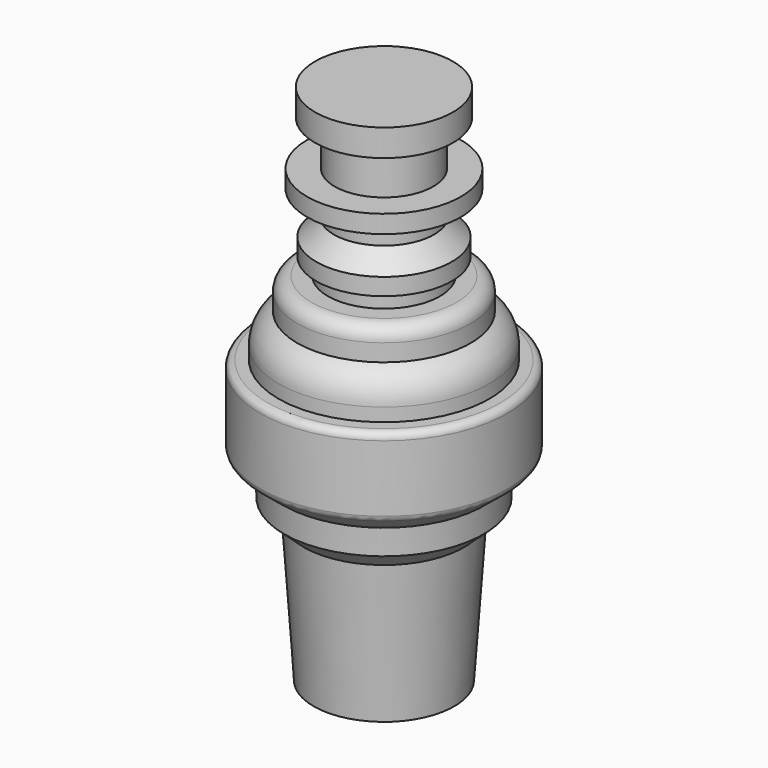
from build123d import *

# Parameters (mm, degrees)
F2_R = 12.7
F4_R = 6.35


# Not quite as in the source:
# - a fillet or chamfer that OpenCascade refuses, or shapes differently, is made with other operations: its cross-section is extruded or revolved along the edge and cut away or added


with BuildPart() as f1:
    # F0 (on Front) → F1 (revolve)
    with BuildSketch(Plane.XZ):
        Polygon((46.7799907497, -259.2296465031), (110.0204106454, -259.2296465031), (110.0204106454, 210.6703534969), (48.0645865742, 210.6703534969), (48.0645865742, 186.4424991518), (65.7015453758, 186.4424991518), (65.7015453758, 146.1238006124), (40.8587217282, 146.1238006124), (40.8587217282, 129.9940093533), (64.9879317765, 129.9940093533), (64.9879317765, 108.3219168065), (49.1057302837, 91.8724802611), (49.1057302837, 76.5575138209), (59.5669516537, 76.5575138209), (59.5669516537, 61.2788777338), (32.0324628472, 61.2788777338), (32.0324628472, 33.1022732576), (15.1265001614, 33.1022732576), (15.1265001614, -5.4745311297), (-1.1045893546, -5.4745311297), (-1.1045893546, -74.4996249259), (19.5996663081, -91.3724261251), (20.3664886729, -114.3807911865), (38.0034474745, -130.4866455729), align=None)
    revolve(axis=Axis((110.0204106454, 0, -24.2796465031), (0, 0, 1)))

    # F2
    f2_edges = [f1.edges().sort_by_distance(p)[0] for p in [
        (188.008358, 0, 61.278878),
    ]]
    fillet(f2_edges, radius=F2_R)

    # F3: fillet of radius 29.4340917525 on 1 edges, made by hand

    # F3_s1 → F3_t2 (revolve, cut)
    with BuildSketch(Plane.XZ):
        with BuildLine():
            ThreePointArc((32.0324628472, 33.1022732576), (19.7098388295, 22.2410689464), (15.1265001614, 6.4674888699))
            Line((15.1265001614, 6.4674888699), (15.1265001614, 33.1022732576))
            Line((15.1265001614, 33.1022732576), (32.0324628472, 33.1022732576))
        make_face()
    revolve(axis=Axis((110.0204106454, 0, 33.1022732576), (0, 0, 1)), mode=Mode.SUBTRACT)

    # F4
    f4_edges = [f1.edges().sort_by_distance(p)[0] for p in [
        (221.145411, 0, -5.474531),
        (221.145411, 0, -74.499625),
    ]]
    fillet(f4_edges, radius=F4_R)


solid = f1.part
